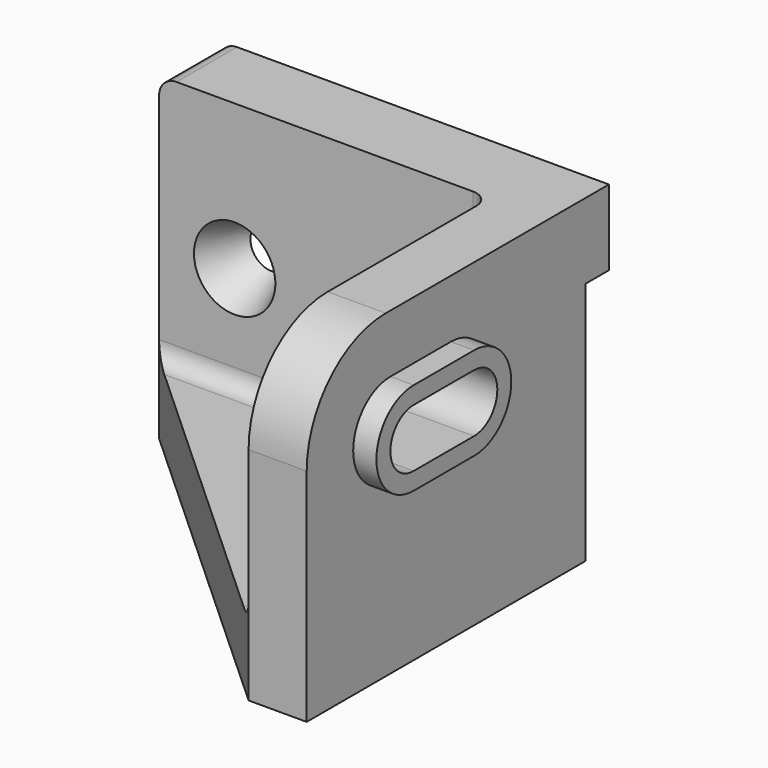
from build123d import *

# Parameters (mm, degrees)
F0_W           = 67
F0_H           = 5
F1_DEPTH       = 12
F2_DEPTH       = 43
F5_DEPTH       = 9
F6_W           = 5
F6_H           = 42
F7_DEPTH       = 100
F9_D           = 5
F9_CSINK_D     = 14
F9_CSINK_ANGLE = 45
F10_R          = 3


# Not quite as in the source:
# - a feature names something its author has since deleted; it is built from what else it names


with BuildPart() as f1:
    # F0 (on Top) → F1 (new body)
    with BuildSketch(Plane.XY):
        Polygon((57, -8), (0, -8), (57, -60), align=None)
        Polygon((67, 0), (0, 0), (0, -8), (57, -8), (57, -60), (67, -60), align=None)
        with Locations((33.5, 2.5)):
            Rectangle(F0_W, F0_H)
    extrude(amount=-F1_DEPTH)

    # F0 (on Top) → F2 (join)
    with BuildSketch(Plane.XY):
        Polygon((67, 0), (0, 0), (0, -8), (57, -8), (57, -60), (67, -60), align=None)
        with Locations((33.5, 2.5)):
            Rectangle(F0_W, F0_H)
    extrude(amount=F2_DEPTH)

    # F4 (on mid) → F5 (join, symmetric)
    with BuildSketch(Plane(origin=(62, 0, 0), x_dir=(0, -1, 0), z_dir=(-1, 0, 0))):
        with BuildLine():
            Line((42, 33), (29, 33))
            ThreePointArc((29, 33), (21, 25), (29, 17))
            Line((29, 17), (42, 17))
            ThreePointArc((42, 17), (50, 25), (42, 33))
        make_face()
        with BuildLine():
            ThreePointArc((42, 30), (47, 25), (42, 20))
            Line((42, 20), (29, 20))
            ThreePointArc((29, 20), (24, 25), (29, 30))
            Line((29, 30), (42, 30))
        make_face(mode=Mode.SUBTRACT)
    extrude(amount=F5_DEPTH, both=True)

    # F6 (on mid) → F7 (cut, symmetric)
    with BuildSketch(Plane(origin=(62, 0, 0), x_dir=(0, -1, 0), z_dir=(-1, 0, 0))):
        with BuildLine():
            ThreePointArc((43, 43), (55.0208152802, 38.0208152802), (60, 26))
            Line((60, 26), (60, 43))
            Line((60, 43), (43, 43))
        make_face()
        with BuildLine():
            Line((42, 30), (29, 30))
            ThreePointArc((29, 30), (24, 25), (29, 20))
            Line((29, 20), (42, 20))
            ThreePointArc((42, 20), (47, 25), (42, 30))
        make_face()
        with Locations((-2.5, 9)):
            Rectangle(F6_W, F6_H)
    extrude(amount=F7_DEPTH, both=True, mode=Mode.SUBTRACT)

    # F9 (through all)
    with Locations(Plane.XZ.offset(8)):
        with Locations((13, 18), (44, 18)):
            CounterSinkHole(F9_D / 2, F9_CSINK_D / 2, counter_sink_angle=F9_CSINK_ANGLE)

    # F10
    f10_edges = [f1.edges().sort_by_distance(p)[0] for p in [
        (57, -21, 25),
        (57, -35.5, 33),
        (57, -34, 0),
        (28.5, -8, 0),
        (57, -8, 21.5),
        (0, -1.5, 43),
    ]]
    fillet(f10_edges, radius=F10_R)


solid = f1.part
